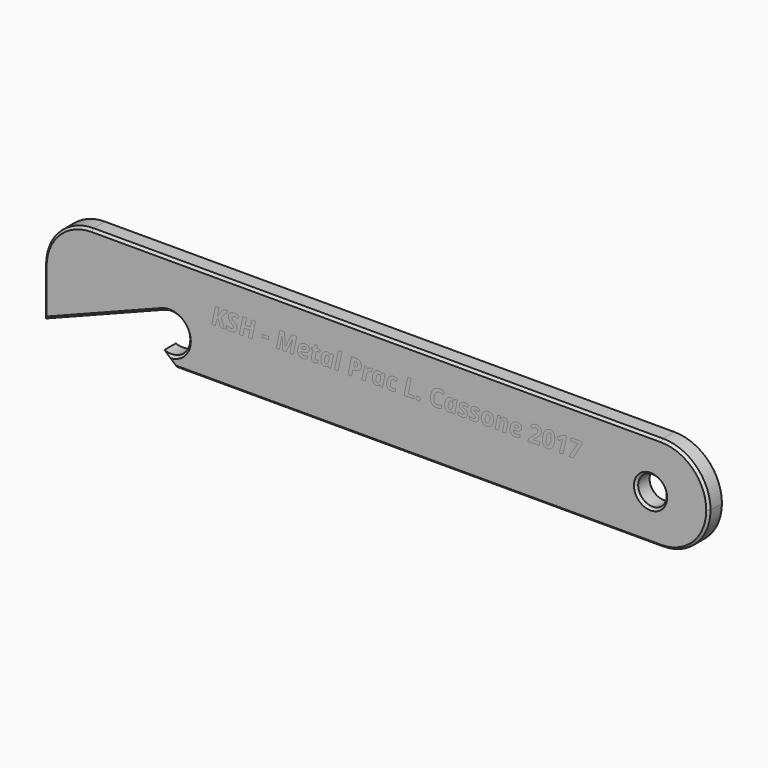
from build123d import *

# Parameters (mm, degrees)
F0_W         = 140
F0_H         = 20
F0_R         = 3
F1_DEPTH     = 4
F3_DEPTH     = 4.001
F4_DEPTH     = 25
F5_DEPTH     = 4.001
F6_C1_SIZE   = 0.5
F6_C2_SIZE   = 0.5
F6_C3_SIZE   = 0.5
F6_C4_SIZE   = 0.5
F6_C5_SIZE   = 0.5
F7_T1_DEPTH  = 7.8768952942
F7_T3_DEPTH  = 103.545799256
F7_T5_DEPTH  = 120
F7_T7_DEPTH  = 27.5171448845
F7_T9_DEPTH  = 10.3692724142
F7_T12_ANGLE = 166.5960015226
F7_T14_ANGLE = 180
F7_T16_ANGLE = 111.307078206
F7_T18_ANGLE = 90
F8_TEXT_SIZE = 5.0497047293
F9_DEPTH     = 1


# Not quite as in the source:
# - a fillet or chamfer that OpenCascade refuses, or shapes differently, is made with other operations: its cross-section is extruded or revolved along the edge and cut away or added
# - Text() gives the source's letters only with a copy of the font that has no kerning and outlines rounded to 1/6400 em; it was checked with that copy


with BuildPart() as f1:
    # F0 (on Front) → F1 (new body)
    with BuildSketch(Plane.XZ):
        with Locations((25.7138942182, -12.0568943769)):
            Rectangle(F0_W, F0_H)
        with Locations((83.4714248776, -12.4128861353)):
            Circle(F0_R, mode=Mode.SUBTRACT)
    extrude(amount=F1_DEPTH)

    # F2 (on face) → F3 (cut, through all)
    with BuildSketch(Plane.XZ.offset(4)):
        with BuildLine():
            ThreePointArc((95.7138942182, -12.0568943769), (92.7849620301, -19.1279621887), (85.7138942182, -22.0568943769))
            Line((85.7138942182, -22.0568943769), (95.7138942182, -22.0568943769))
            Line((95.7138942182, -22.0568943769), (95.7138942182, -12.0568943769))
        make_face()
        with BuildLine():
            ThreePointArc((85.7138942182, -2.0568943769), (92.7849620301, -4.985826565), (95.7138942182, -12.0568943769))
            Line((95.7138942182, -12.0568943769), (95.7138942182, -2.0568943769))
            Line((95.7138942182, -2.0568943769), (85.7138942182, -2.0568943769))
        make_face()
        with BuildLine():
            ThreePointArc((-44.2861057818, -12.0568943769), (-41.3571735937, -4.985826565), (-34.2861057818, -2.0568943769))
            Line((-34.2861057818, -2.0568943769), (-44.2861057818, -2.0568943769))
            Line((-44.2861057818, -2.0568943769), (-44.2861057818, -12.0568943769))
        make_face()
    extrude(amount=-F3_DEPTH, mode=Mode.SUBTRACT)

    # F2 (on face) → F4 (cut)
    with BuildSketch(Plane.XZ.offset(4)):
        with BuildLine():
            Line((-44.2861057818, -22.0568943769), (-16.6811272502, -22.0568943769))
            Line((-16.6811272502, -22.0568943769), (-19.3478078496, -19.7834797575))
            ThreePointArc((-19.3478078496, -19.7834797575), (-21.8943425417, -16.0568943769), (-19.3478078496, -12.3303089963))
            Line((-19.3478078496, -12.3303089963), (-44.2861057818, -22.0568943769))
        make_face()
    extrude(amount=-F4_DEPTH, mode=Mode.SUBTRACT)

    # F2 (on face) → F5 (cut, through all)
    with BuildSketch(Plane.XZ.offset(4)):
        with BuildLine():
            ThreePointArc((-19.3478078496, -12.3303089963), (-21.8943425417, -16.0568943769), (-19.3478078496, -19.7834797575))
            ThreePointArc((-19.3478078496, -19.7834797575), (-15.6375595694, -19.3594586254), (-13.8943425417, -16.0568943769))
            ThreePointArc((-13.8943425417, -16.0568943769), (-15.6375595694, -12.7543301283), (-19.3478078496, -12.3303089963))
        make_face()
    extrude(amount=-F5_DEPTH, mode=Mode.SUBTRACT)

    # F6: chamfer of 0.5 on 11 edges, made by hand

    # F6_c1
    f6_c1_edges = [f1.edges().sort_by_distance(p)[0] for p in [
        (25.7138942182, 0, -2.0568943769),
        (95.7138942182, 0, -12.0568943769),
        (34.516383484, 0, -22.0568943769),
        (-44.2861057818, 0, -17.0568943769),
        (-41.3571735937, 0, -4.985826565),
    ]]
    chamfer(f6_c1_edges, length=F6_C1_SIZE)

    # F6_c2
    f6_c2_edges = [f1.edges().sort_by_distance(p)[0] for p in [
        (25.7138942182, -4, -2.0568943769),
        (-41.3571735937, -4, -4.985826565),
        (-44.2861057818, -4, -17.0568943769),
        (95.7138942182, -4, -12.0568943769),
        (34.516383484, -4, -22.0568943769),
    ]]
    chamfer(f6_c2_edges, length=F6_C2_SIZE)

    # F6_c3
    f6_c3_edges = [f1.edges().sort_by_distance(p)[0] for p in [
        (-18.3077137286, -4, -20.6701870672),
    ]]
    chamfer(f6_c3_edges, length=F6_C3_SIZE)

    # F6_c4
    f6_c4_edges = [f1.edges().sort_by_distance(p)[0] for p in [
        (-15.2049906997, -4, -19.0178716935),
        (-15.6375595694, -4, -12.7543301283),
        (-31.5669568157, -4, -17.0960951787),
    ]]
    chamfer(f6_c4_edges, length=F6_C4_SIZE)

    # F6_c5
    f6_c5_edges = [f1.edges().sort_by_distance(p)[0] for p in [
        (80.4714248776, -4, -12.4128861353),
    ]]
    chamfer(f6_c5_edges, length=F6_C5_SIZE)

    # F7: chamfer of 0.5 on 10 edges, made by hand

    # F7_s2 → F7_t1 (cut)
    with BuildSketch(Plane(origin=(1.6214319868, 0, -1.3823129715), x_dir=(0, 1, 0), z_dir=(-0.7609899144, 0, 0.6487637091))):
        Polygon((-0.5, 27.6071841497), (0, 27.1071841497), (0, 27.6071841497), align=None)
    extrude(amount=F7_T1_DEPTH, mode=Mode.SUBTRACT)

    # F7_s4 → F7_t3 (cut)
    with BuildSketch(Plane.YZ.offset(-17.8319050378)):
        Polygon((0, -21.3497875957), (-0.1464466094, -21.7033409863), (0, -21.5568943769), align=None)
    extrude(amount=F7_T3_DEPTH, mode=Mode.SUBTRACT)

    # F7_s6 → F7_t5 (cut)
    with BuildSketch(Plane.YZ.offset(-34.2861057818)):
        Polygon((0, -2.7640011581), (-0.1464466094, -2.4104477675), (0, -2.5568943769), align=None)
    extrude(amount=F7_T5_DEPTH, mode=Mode.SUBTRACT)

    # F7_s8 → F7_t7 (cut)
    with BuildSketch(Plane(origin=(-20.967384416, 0, -8.1778257395), x_dir=(0, 1, 0), z_dir=(-0.9316463451, 0, -0.363366327))):
        Polygon((-0.5, 4.4571454376), (0, 3.9571454376), (0, 4.4571454376), align=None)
    extrude(amount=F7_T7_DEPTH, mode=Mode.SUBTRACT)

    # F7_s10 → F7_t9 (cut)
    with BuildSketch(Plane.XY.offset(-22.4261667911)):
        Polygon((-43.5789990006, 0), (-43.9325523912, -0.1464466094), (-43.7861057818, 0), align=None)
    extrude(amount=F7_T9_DEPTH, mode=Mode.SUBTRACT)

    # F7_s11 → F7_t12 (revolve, cut)
    with BuildSketch(Plane(origin=(2.6592304748, 0, -11.1588268023), x_dir=(0, 1, 0), z_dir=(-0.2318157896, 0, 0.9727597029))):
        Polygon((-0.5, 25.1291369845), (0, 25.6291369845), (0, 25.1291369845), align=None)
    revolve(axis=Axis((-17.8943425417, 0, -16.0568943769), (0, -1, 0)), revolution_arc=F7_T12_ANGLE, mode=Mode.SUBTRACT)

    # F7_s13 → F7_t14 (revolve, cut)
    with BuildSketch(Plane.YZ.offset(85.7138942182)):
        Polygon((0, -21.3497875957), (-0.1464466094, -21.7033409863), (0, -21.5568943769), align=None)
    revolve(axis=Axis((85.7138942182, 0, -12.0568943769), (0, -1, 0)), revolution_arc=F7_T14_ANGLE, mode=Mode.SUBTRACT)

    # F7_s15 → F7_t16 (revolve, cut)
    with BuildSketch(Plane.XY.offset(-16.0568943769)):
        Polygon((-13.8943425417, -0.5), (-13.3943425417, 0), (-13.8943425417, 0), align=None)
    revolve(axis=Axis((-17.8943425417, 0, -16.0568943769), (0, -1, 0)), revolution_arc=F7_T16_ANGLE, mode=Mode.SUBTRACT)

    # F7_s17 → F7_t18 (revolve, cut)
    with BuildSketch(Plane.YZ.offset(-34.2861057818)):
        Polygon((0, -2.7640011581), (-0.1464466094, -2.4104477675), (0, -2.5568943769), align=None)
    revolve(axis=Axis((-34.2861057818, 0, -12.0568943769), (0, -1, 0)), revolution_arc=F7_T18_ANGLE, mode=Mode.SUBTRACT)

    # F7_s19 → F7_t20 (revolve, cut)
    with BuildSketch(Plane.XY.offset(-12.4128861353)):
        Polygon((86.4714248776, -0.5), (86.9714248776, 0), (86.4714248776, 0), align=None)
    revolve(axis=Axis((83.4714248776, 0, -12.4128861353), (0, -1, 0)), mode=Mode.SUBTRACT)


with BuildPart() as f9:
    # F8 (on face) → F9 (new body)
    with BuildSketch(Plane.XZ.offset(4)):
        with Locations((-9.0921586379, -11.471808888)):
            Text('KSH - Metal Prac L. Cassone 2017', F8_TEXT_SIZE, font='Open Sans', font_style=FontStyle.BOLDITALIC, text_align=(TextAlign.LEFT, TextAlign.BOTTOM))
    extrude(amount=-F9_DEPTH)


solid = Compound([f1.part, f9.part])
